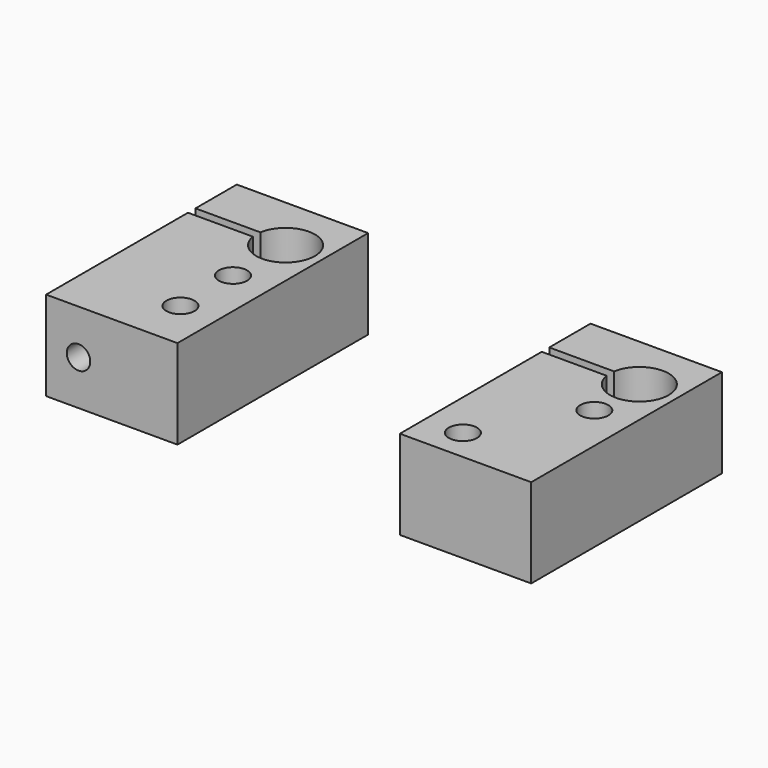
from build123d import *

# Parameters (mm, degrees)
F0_R     = 1.5
F1_DEPTH = 9.525
F2_R     = 1.25
F3_DEPTH = 25.401
F4_R     = 1.5
F5_DEPTH = 9.5
F6_R     = 1.6
F7_DEPTH = 20


# Not quite as in the source:
# - a length typed as a fraction of an inch, garbled in the dataset ("3 / 203.2 mm" for 3/8 in), is restored


with BuildPart() as f1:
    # F0 (on Top) → F1 (new body)
    with BuildSketch(Plane.XY):
        with BuildLine():
            Line((-7, -12.7), (7, -12.7))
            Line((7, -12.7), (7, 12.7))
            Line((7, 12.7), (-7, 12.7))
            Line((-7, 12.7), (-7, 7.2))
            Line((-7, 7.2), (-0.0847406698, 7.2))
            ThreePointArc((-0.0847406698, 7.2), (6.125, 6.7), (-0.0847406698, 6.2))
            Line((-0.0847406698, 6.2), (-7, 6.2))
            Line((-7, 6.2), (-7, -12.7))
        make_face()
        with Locations((3, -7.3)):
            Circle(F0_R, mode=Mode.SUBTRACT)
        with Locations((3, -0.3)):
            Circle(F0_R, mode=Mode.SUBTRACT)
    extrude(amount=F1_DEPTH)

    # F2 (on face) → F3 (cut, through all)
    with BuildSketch(Plane(origin=(0, 12.7, 0), x_dir=(-1, 0, 0), z_dir=(0, 1, 0))):
        with Locations((3.5423703349, 4.7625)):
            Circle(F2_R)
    extrude(amount=-F3_DEPTH, mode=Mode.SUBTRACT)


with BuildPart() as f5:
    # F4 (on Top) → F5 (new body)
    with BuildSketch(Plane.XY):
        with BuildLine():
            Line((31.6146114171, -13.843855077), (45.6146114171, -13.843855077))
            Line((45.6146114171, -13.843855077), (45.6146114171, 11.556144923))
            Line((45.6146114171, 11.556144923), (31.6146114171, 11.556144923))
            Line((31.6146114171, 11.556144923), (31.6146114171, 6.056144923))
            Line((31.6146114171, 6.056144923), (38.5298707472, 6.056144923))
            ThreePointArc((38.5298707472, 6.056144923), (44.7396114171, 5.556144923), (38.5298707472, 5.056144923))
            Line((38.5298707472, 5.056144923), (31.6146114171, 5.056144923))
            Line((31.6146114171, 5.056144923), (31.6146114171, -13.843855077))
        make_face()
        with Locations((35.6146114171, -10.443855077)):
            Circle(F4_R, mode=Mode.SUBTRACT)
        with Locations((41.6146114171, -0.443855077)):
            Circle(F4_R, mode=Mode.SUBTRACT)
    extrude(amount=F5_DEPTH)

    # F6 (on face) → F7 (cut)
    with BuildSketch(Plane(origin=(0, 11.556144923, 0), x_dir=(-1, 0, 0), z_dir=(0, 1, 0))):
        with Locations((-35.0722410821, 4.75)):
            Circle(F6_R)
    extrude(amount=-F7_DEPTH, mode=Mode.SUBTRACT)


solid = Compound([f1.part, f5.part])
